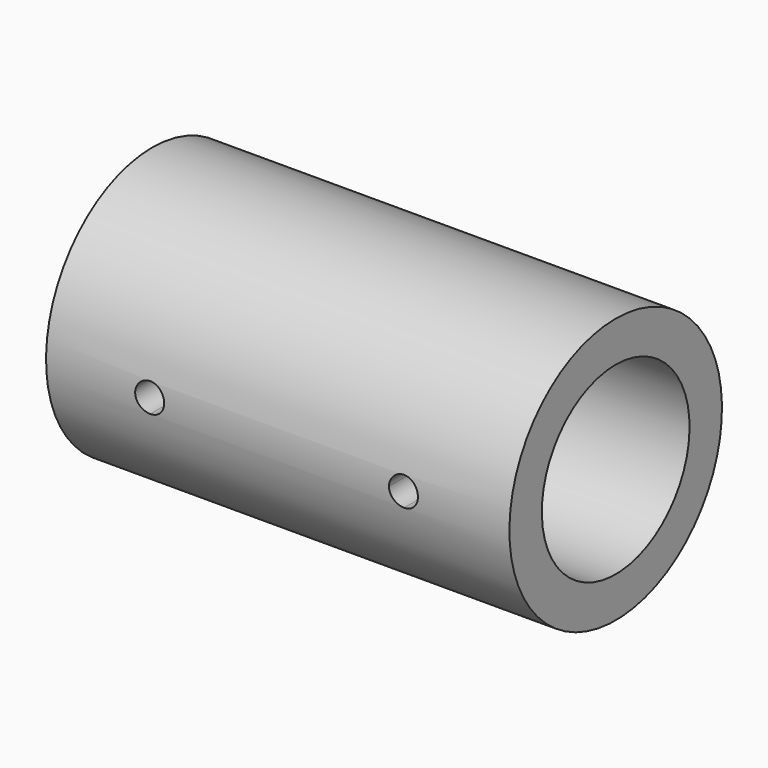
from build123d import *

# Parameters (mm, degrees)
F0_W     = 160
F0_H     = 14
F3_DEPTH = 45.8700225313


# Not quite as in the source:
# - the program builds the solid bodies; features that only make, move or delete a surface that nothing else refers to are left out


with BuildPart() as f1:
    # F0 (on Front) → F1 (revolve)
    with BuildSketch(Plane.XZ):
        with Locations((0.4038456827, 38.8690225313)):
            Rectangle(F0_W, F0_H)
    revolve(axis=Axis((59.6884675324, 0, 0), (1, 0, 0)))

    # F2 (on Front) → F3 (cut, through all)
    with BuildSketch(Plane.XZ):
        with BuildLine():
            ThreePointArc((-38.8187138988, 0), (-40.2831799929, 3.5355339059), (-43.8187138988, 5))
            Line((-43.8187138988, 5), (-43.8187138988, -5))
            ThreePointArc((-43.8187138988, -5), (-40.2831799929, -3.5355339059), (-38.8187138988, 0))
        make_face()
        with BuildLine():
            Line((-43.8187138988, -5), (-43.8187138988, 5))
            ThreePointArc((-43.8187138988, 5), (-48.8187138988, 0), (-43.8187138988, -5))
        make_face()
    f3 = extrude(amount=F3_DEPTH, mode=Mode.SUBTRACT)

    # F4: F3 across plane
    add(f3.mirror(Plane.YZ), mode=Mode.SUBTRACT)


solid = f1.part
